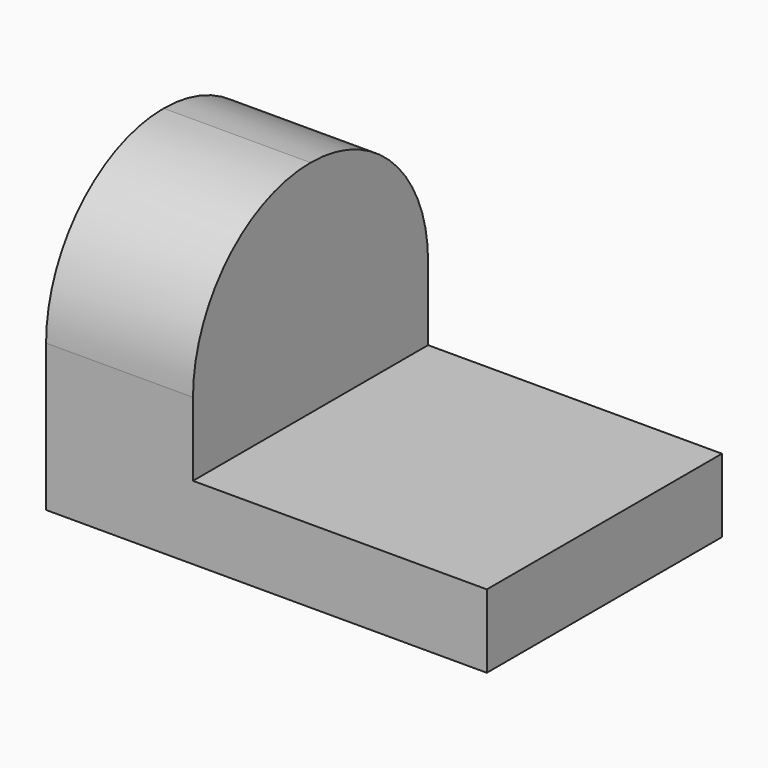
from build123d import *

# Parameters (mm, degrees)
F1_DEPTH = 25.4
F2_R     = 12.69999


# Not quite as in the source:
# - a fillet or chamfer is up to 0.001 mm smaller than in the source, because OpenCascade refuses the exact size


with BuildPart() as f1:
    # F0 (on Front) → F1 (new body)
    with BuildSketch(Plane.XZ):
        Polygon((-3.4890425639, 19.6637109485), (-16.1890425639, 19.6637109485), (-16.1890425639, -5.7362890515), (21.9109574361, -5.7362890515), (21.9109574361, 0.6137109485), (-3.4890425639, 0.6137109485), align=None)
    extrude(amount=F1_DEPTH)

    # F2 (radius 12.7 in the source; OpenCascade refuses exactly that, so slightly less here)
    f2_edges = [f1.edges().sort_by_distance(p)[0] for p in [
        (-9.839043, -25.4, 19.663711),
        (-9.839043, 0, 19.663711),
    ]]
    fillet(f2_edges, radius=F2_R)


solid = f1.part
